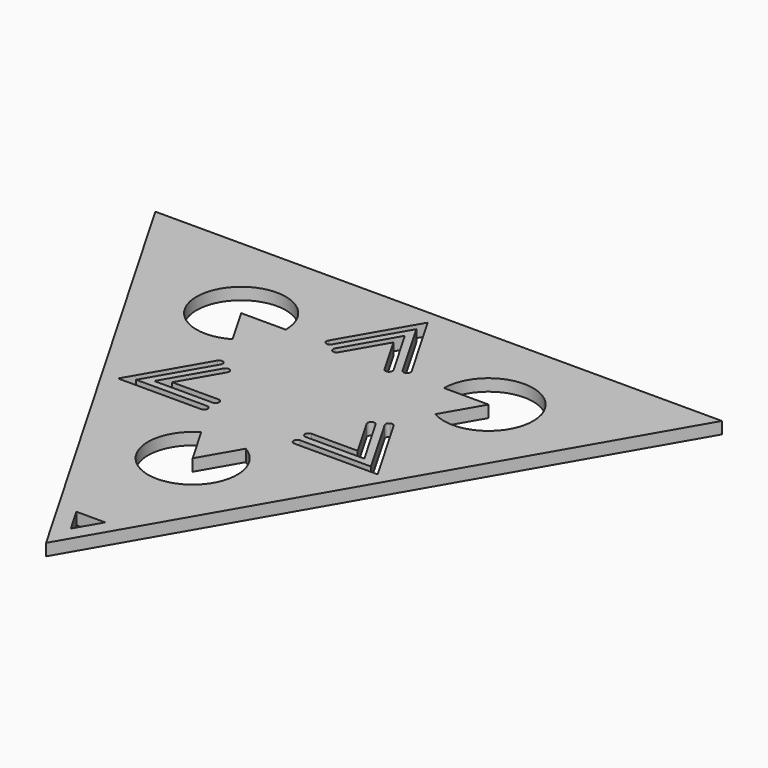
from build123d import *

# Parameters (mm, degrees)
F1_DEPTH = 1.27


# Not quite as in the source:
# - a feature of the source that left no trace in its solid (it failed there, or was rolled back) is left out


with BuildPart() as f1:
    # F0 (on Top) → F1 (new body)
    with BuildSketch(Plane.XY):
        Polygon((30.2459372272, 16.8275), (-30.2459372272, 16.8275), (0, -35.56), align=None)
        Polygon((-1.5397931679, -29.591), (1.5397931679, -29.591), (0, -32.258), align=None, mode=Mode.SUBTRACT)
        with BuildLine():
            ThreePointArc((2.38125, -11.8775540145), (0, -20.7645), (-2.38125, -11.8775540145))
            Line((-2.38125, -11.8775540145), (0, -16.002))
            Line((0, -16.002), (2.38125, -11.8775540145))
        make_face(mode=Mode.SUBTRACT)
        with BuildLine():
            Line((-8.7532271537, -1.3180341604), (-12.538315796, -7.874))
            Line((-12.538315796, -7.874), (-4.9681385114, -7.874))
            ThreePointArc((-4.9681385114, -7.874), (-4.6987308277, -7.9855923164), (-4.5871385114, -8.255))
            ThreePointArc((-4.5871385114, -8.255), (-4.6987308277, -8.5244076836), (-4.9681385114, -8.636))
            Line((-4.9681385114, -8.636), (-13.8581385114, -8.636))
            Line((-13.8581385114, -8.636), (-9.4131385114, -0.9370341604))
            ThreePointArc((-9.4131385114, -0.9370341604), (-9.1817928887, -0.7595164205), (-8.8926828325, -0.7975784815))
            ThreePointArc((-8.8926828325, -0.7975784815), (-8.7151650927, -1.0289241042), (-8.7532271537, -1.3180341604))
        make_face(mode=Mode.SUBTRACT)
        with BuildLine():
            Line((-4.9681385114, -7.112), (-11.2184930806, -7.112))
            Line((-11.2184930806, -7.112), (-8.093315796, -1.6990341604))
            ThreePointArc((-8.093315796, -1.6990341604), (-7.5728601171, -1.5595784815), (-7.4334044383, -2.0800341604))
            Line((-7.4334044383, -2.0800341604), (-9.8986703653, -6.35))
            Line((-9.8986703653, -6.35), (-4.9681385114, -6.35))
            ThreePointArc((-4.9681385114, -6.35), (-4.5871385114, -6.731), (-4.9681385114, -7.112))
        make_face(mode=Mode.SUBTRACT)
        with BuildLine():
            ThreePointArc((-10.82675, 2.8605540145), (-17.3324459855, 9.36625), (-8.4455, 6.985))
            Line((-8.4455, 6.985), (-13.208, 6.985))
            Line((-13.208, 6.985), (-10.82675, 2.8605540145))
        make_face(mode=Mode.SUBTRACT)
        with BuildLine():
            Line((4.9681385114, -7.874), (12.538315796, -7.874))
            Line((12.538315796, -7.874), (8.7532271537, -1.3180341604))
            ThreePointArc((8.7532271537, -1.3180341604), (8.7151650927, -1.0289241042), (8.8926828325, -0.7975784815))
            ThreePointArc((8.8926828325, -0.7975784815), (9.1817928887, -0.7595164205), (9.4131385114, -0.9370341604))
            Line((9.4131385114, -0.9370341604), (13.8581385114, -8.636))
            Line((13.8581385114, -8.636), (4.9681385114, -8.636))
            ThreePointArc((4.9681385114, -8.636), (4.6987308277, -8.5244076836), (4.5871385114, -8.255))
            ThreePointArc((4.5871385114, -8.255), (4.6987308277, -7.9855923164), (4.9681385114, -7.874))
        make_face(mode=Mode.SUBTRACT)
        with BuildLine():
            Line((4.9681385114, -6.35), (9.8986703653, -6.35))
            Line((9.8986703653, -6.35), (7.4334044383, -2.0800341604))
            ThreePointArc((7.4334044383, -2.0800341604), (7.5728601171, -1.5595784815), (8.093315796, -1.6990341604))
            Line((8.093315796, -1.6990341604), (11.2184930806, -7.112))
            Line((11.2184930806, -7.112), (4.9681385114, -7.112))
            ThreePointArc((4.9681385114, -7.112), (4.5871385114, -6.731), (4.9681385114, -6.35))
        make_face(mode=Mode.SUBTRACT)
        with BuildLine():
            Line((-3.1251772846, 6.9060341604), (0, 12.319))
            Line((0, 12.319), (3.1251772846, 6.9060341604))
            ThreePointArc((3.1251772846, 6.9060341604), (2.9857216058, 6.3855784815), (2.4652659269, 6.5250341604))
            Line((2.4652659269, 6.5250341604), (0, 10.795))
            Line((0, 10.795), (-2.4652659269, 6.5250341604))
            ThreePointArc((-2.4652659269, 6.5250341604), (-2.9857216058, 6.3855784815), (-3.1251772846, 6.9060341604))
        make_face(mode=Mode.SUBTRACT)
        with BuildLine():
            ThreePointArc((8.4455, 6.985), (17.3324459855, 9.36625), (10.82675, 2.8605540145))
            Line((10.82675, 2.8605540145), (13.208, 6.985))
            Line((13.208, 6.985), (8.4455, 6.985))
        make_face(mode=Mode.SUBTRACT)
        with BuildLine():
            Line((3.7850886423, 7.2870341604), (0, 13.843))
            Line((0, 13.843), (-3.7850886423, 7.2870341604))
            ThreePointArc((-3.7850886423, 7.2870341604), (-4.016434265, 7.1095164205), (-4.3055443212, 7.1475784815))
            ThreePointArc((-4.3055443212, 7.1475784815), (-4.483062061, 7.3789241042), (-4.445, 7.6680341604))
            Line((-4.445, 7.6680341604), (0, 15.367))
            Line((0, 15.367), (4.445, 7.6680341604))
            ThreePointArc((4.445, 7.6680341604), (4.483062061, 7.3789241042), (4.3055443212, 7.1475784815))
            ThreePointArc((4.3055443212, 7.1475784815), (4.016434265, 7.1095164205), (3.7850886423, 7.2870341604))
        make_face(mode=Mode.SUBTRACT)
    extrude(amount=F1_DEPTH)


solid = f1.part
